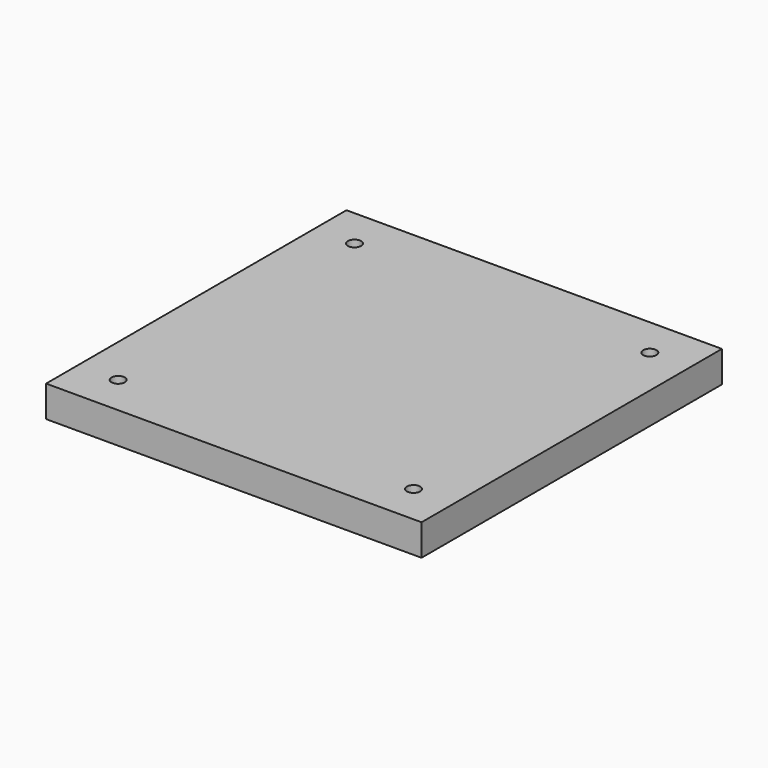
from build123d import *

# Parameters (mm, degrees)
F0_W     = 76.2
F0_H     = 76.2
F1_DEPTH = 6.35
F3_D     = 2.7051


with BuildPart() as f1:
    # F0 (on Top) → F1 (new body)
    with BuildSketch(Plane.XY):
        Rectangle(F0_W, F0_H)
    extrude(amount=F1_DEPTH)

    # F3 (through all)
    with Locations(Plane.XY.offset(6.35)):
        with Locations((-29.972, 29.972), (29.972, 29.972), (29.972, -29.972), (-29.972, -29.972)):
            Hole(F3_D / 2)


solid = f1.part
